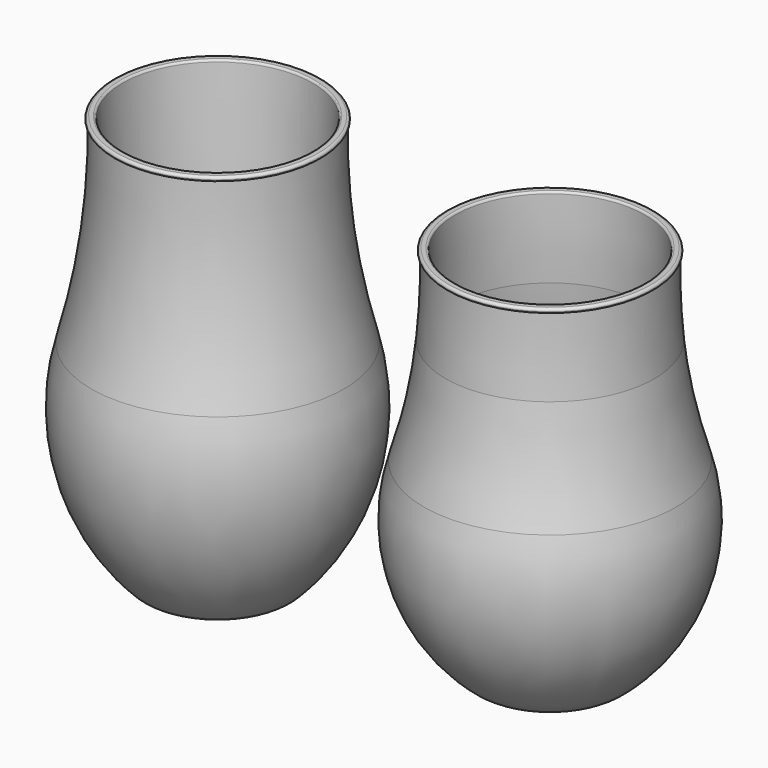
from build123d import *

# Parameters (mm, degrees)
F3_R      = 125.9850186155
F4_DEPTH  = 30
F12_R     = 66.2325488452
F13_DEPTH = 35


# Not quite as in the source:
# - ends of sketch curves that miss each other by under 0.0002 mm in the source are joined


with BuildPart() as f2:
    # F1 (on Front) → F2 (revolve)
    with BuildSketch(Plane.XZ):
        with BuildLine():
            ThreePointArc((-27.8148734311, 59.4126989909), (-29.3430504586, 29.9739316777), (-35.1395822774, 1.0710500771))
            ThreePointArc((-35.1395822774, 1.0710500771), (-35.4177932294, -30.0336371057), (-20.0947995033, -57.1036355115))
            ThreePointArc((-20.0947995033, -57.1036355115), (-19.1154867702, -57.7668490394), (-17.955941, -58))
            Line((-17.955941, -58), (-15.394804, -58))
            ThreePointArc((-15.394804, -58), (-7.8421934259, -55.7569881561), (0, -55))
            Line((0, -55), (0, 60))
            Line((0, 60), (-28.414739, 60))
            ThreePointArc((-28.414739, 60), (-27.9949887141, 59.8287303318), (-27.8148734311, 59.4126989909))
        make_face()
    revolve(axis=Axis((0, 0, 2.5), (0, 0, 1)))

    # F3 (on face) → F4 (cut)
    with BuildSketch(Plane.XY.offset(60)):
        Circle(F3_R)
    extrude(amount=-F4_DEPTH, mode=Mode.SUBTRACT)


with BuildPart() as f6:
    # F5 (on Front) → F6 (revolve)
    with BuildSketch(Plane.XZ):
        with BuildLine():
            ThreePointArc((-35.1395822774, 1.0710500771), (-29.3430504586, 29.9739316777), (-27.8148734311, 59.4126989909))
            ThreePointArc((-27.8148734311, 59.4126989909), (-27.9949887141, 59.8287303318), (-28.414739, 60))
            Line((-28.414739, 60), (-29.548, 60))
            ThreePointArc((-29.548, 60), (-30.0783300859, 59.7803300859), (-30.298, 59.25))
            ThreePointArc((-30.298, 59.25), (-30.1571169652, 58.8637208104), (-29.800627959, 58.6588422359))
            ThreePointArc((-29.800627959, 58.6588422359), (-31.3721118802, 29.8700547766), (-37.0666121939, 1.6063590539))
            ThreePointArc((-37.0666121939, 1.6063590539), (-37.3540901939, -30.5343906031), (-21.5207043341, -58.506060345))
            ThreePointArc((-21.5207043341, -58.506060345), (-19.8885166315, -59.611415339), (-17.955941, -60))
            Line((-17.955941, -60), (-15, -60))
            ThreePointArc((-15, -60), (-9.1733292762, -58.0941952995), (-3.119996, -57.1250000005))
            ThreePointArc((-3.119996, -57.1250000005), (-1.6201851772, -57.7771100034), (0, -58))
            Line((0, -58), (0, -55))
            ThreePointArc((0, -55), (-7.8421934259, -55.7569881561), (-15.3948040449, -57.9999998892))
            Line((-15.3948040449, -57.9999998892), (-17.955941, -58))
            ThreePointArc((-17.955941, -58), (-19.1154867702, -57.7668490394), (-20.0947997335, -57.1036357379))
            ThreePointArc((-20.0947997335, -57.1036357379), (-35.4177932294, -30.0336371057), (-35.1395822774, 1.0710500771))
        make_face()
    revolve(axis=Axis((0, 0, -56.5), (0, 0, 1)))


with BuildPart() as f8:
    # F7 (on Front) → F8 (revolve)
    with BuildSketch(Plane.XZ):
        with BuildLine():
            Line((-23.1621605088, -29.3663516937), (-27.814873402, 59.4126989915))
            ThreePointArc((-27.814873402, 59.4126989915), (-27.9949887141, 59.8287303318), (-28.414739, 60))
            Line((-28.414739, 60), (-29.548, 60))
            ThreePointArc((-29.548, 60), (-30.0783300859, 59.7803300859), (-30.298, 59.25))
            ThreePointArc((-30.298, 59.25), (-30.1571169652, 58.8637208104), (-29.800627959, 58.6588422359))
            Line((-29.800627959, 58.6588422359), (-26.6924057931, -30.348994967))
            ThreePointArc((-26.6924057931, -30.348994967), (-23.6450812275, -37.1933980034), (-16.6984975229, -40))
            Line((-16.6984975229, -40), (-2.8397459622, -40))
            Line((-2.8397459622, -40), (-1.5, -45))
            Line((-1.5, -45), (0, -45))
            Line((0, -45), (0, -40))
            Line((0, -40), (0, -36))
            Line((0, -36), (-16.1717537655, -36))
            ThreePointArc((-16.1717537655, -36), (-20.9902357953, -34.0776205971), (-23.1621605088, -29.3663516937))
        make_face()
    revolve(axis=Axis((0, 0, -38), (0, 0, 1)))


with BuildPart() as f11:
    # F10 (on Front) → F11 (revolve)
    with BuildSketch(Plane.XZ):
        with BuildLine():
            ThreePointArc((68.999728, 57.675086), (69.4194779288, 57.5038166816), (69.5995935768, 57.087785991))
            ThreePointArc((69.5995935768, 57.087785991), (69.5074708351, 45.3637455867), (68.7353078746, 33.6647980119))
            ThreePointArc((68.7353078746, 33.6647980119), (66.3650176206, 17.7529077236), (62.3262707654, 2.1806550743))
            ThreePointArc((62.3262707654, 2.1806550743), (62.1123827267, -26.1369657711), (77.8854656516, -49.65596343))
            ThreePointArc((77.8854656516, -49.65596343), (78.7721946927, -50.1527355037), (79.773906, -50.324914))
            Line((79.773906, -50.324914), (82.019662, -50.324914))
            ThreePointArc((82.019662, -50.324914), (89.5722731193, -48.0819022447), (97.414467, -47.324914))
            Line((97.414467, -47.324914), (97.414467, 57.675086))
            Line((97.414467, 57.675086), (68.999728, 57.675086))
        make_face()
    revolve(axis=Axis((97.414467, 0, 5.175086), (0, 0, -1)))

    # F12 (on face) → F13 (cut)
    with BuildSketch(Plane.XY.offset(57.675086)):
        with Locations((97.414467, 0)):
            Circle(F12_R)
    extrude(amount=-F13_DEPTH, mode=Mode.SUBTRACT)


with BuildPart() as f15:
    # F14 (on Front) → F15 (revolve)
    with BuildSketch(Plane.XZ):
        with BuildLine():
            ThreePointArc((68.7353078746, 33.6647980119), (69.5074708351, 45.3637455867), (69.5995935689, 57.0877859909))
            ThreePointArc((69.5995935689, 57.0877859909), (69.4194779288, 57.5038166816), (68.999728, 57.675086))
            Line((68.999728, 57.675086), (67.866467, 57.675086))
            ThreePointArc((67.866467, 57.675086), (67.3361369141, 57.4554160859), (67.116467, 56.925086))
            ThreePointArc((67.116467, 56.925086), (67.2573499798, 56.5388068759), (67.6138388724, 56.3339282652))
            ThreePointArc((67.6138388724, 56.3339282652), (67.4953938268, 45.0819176273), (66.7443132039, 33.8543770758))
            ThreePointArc((66.7443132039, 33.8543770758), (64.4052109803, 18.1518537511), (60.4196055267, 2.7844991499))
            ThreePointArc((60.4196055267, 2.7844991499), (60.1968137028, -26.7119399572), (76.6265054701, -51.2099966541))
            ThreePointArc((76.6265054701, -51.2099966541), (78.1043872534, -52.0379498746), (79.773906, -52.324914))
            Line((79.773906, -52.324914), (82.414467, -52.324914))
            ThreePointArc((82.414467, -52.324914), (88.2411377238, -50.4191092995), (94.294471, -49.4499140005))
            ThreePointArc((94.294471, -49.4499140005), (95.7942818228, -50.1020240034), (97.414467, -50.324914))
            Line((97.414467, -50.324914), (97.414467, -47.324914))
            ThreePointArc((97.414467, -47.324914), (89.5722731193, -48.0819022447), (82.0196620961, -50.3249142372))
            Line((82.0196620961, -50.3249142372), (79.773906, -50.324914))
            ThreePointArc((79.773906, -50.324914), (78.7721946927, -50.1527355037), (77.8854654832, -49.6559636379))
            ThreePointArc((77.8854654832, -49.6559636379), (62.1123827267, -26.1369657711), (62.3262709137, 2.1806550273))
            ThreePointArc((62.3262709137, 2.1806550273), (66.3650176206, 17.7529077236), (68.7353078746, 33.6647980119))
        make_face()
    revolve(axis=Axis((97.414467, 0, -48.824914), (0, 0, -1)))


solid = Compound([f2.part, f6.part, f8.part, f11.part, f15.part])
